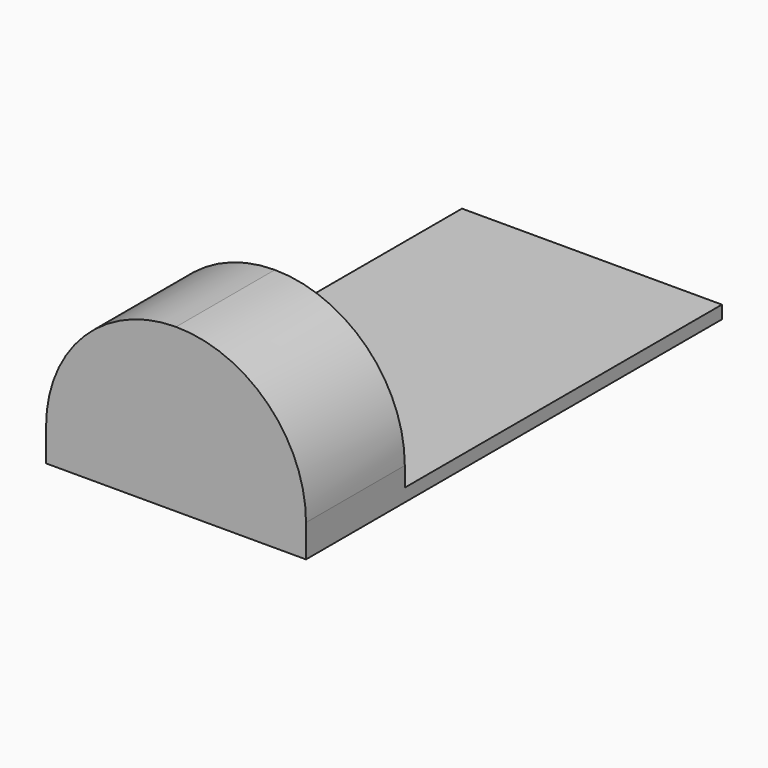
from build123d import *

# Parameters (mm, degrees)
F0_W     = 40
F0_H     = 61
F1_DEPTH = 2
F0_H_2   = 19
F2_DEPTH = 25
F3_R     = 8.5
F4_DEPTH = 17
F5_R     = 19.99999


# Not quite as in the source:
# - a fillet or chamfer is up to 0.001 mm smaller than in the source, because OpenCascade refuses the exact size


with BuildPart() as f1:
    # F0 (on Top) → F1 (new body)
    with BuildSketch(Plane.XY):
        with Locations((-2.8480109572, 28.6193176061)):
            Rectangle(F0_W, F0_H)
    extrude(amount=F1_DEPTH)

    # F0 (on Top) → F2 (join)
    with BuildSketch(Plane.XY):
        with Locations((-2.8480109572, -11.3806823939)):
            Rectangle(F0_W, F0_H_2)
    extrude(amount=F2_DEPTH)

    # F3 (on face) → F4 (cut)
    with BuildSketch(Plane(origin=(0, -1.8806823939, 0), x_dir=(-1, 0, 0), z_dir=(0, 1, 0))):
        with Locations((2.8480109572, 13.5)):
            Circle(F3_R)
    extrude(amount=-F4_DEPTH, mode=Mode.SUBTRACT)

    # F5 (radius 20 in the source; OpenCascade refuses exactly that, so slightly less here)
    f5_edges = [f1.edges().sort_by_distance(p)[0] for p in [
        (17.151989, -11.380682, 25),
        (-22.848011, -11.380682, 25),
    ]]
    fillet(f5_edges, radius=F5_R)


solid = f1.part
